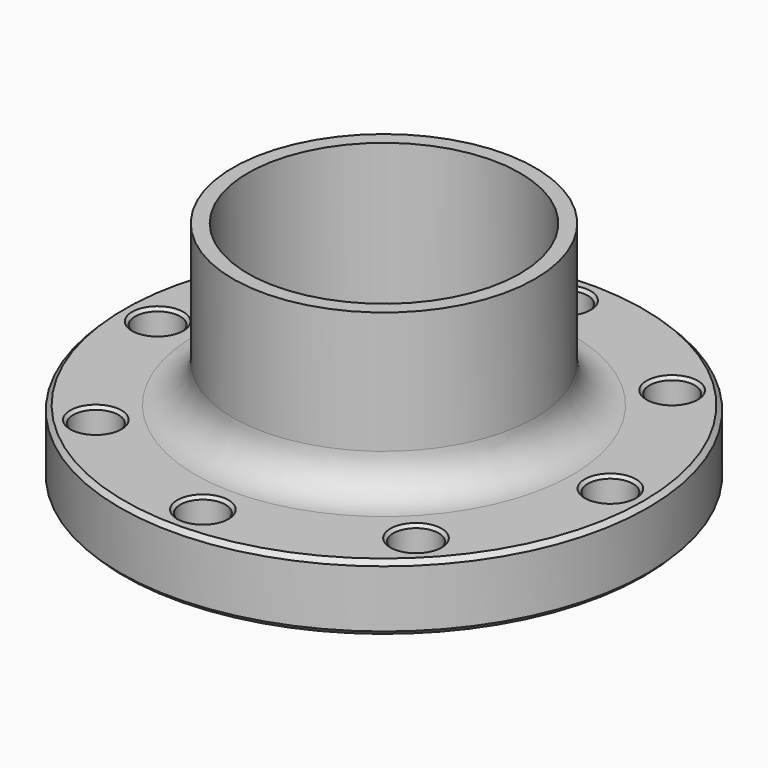
from build123d import *

# Parameters (mm, degrees)
F3_D            = 3.81
F3_CSINK_D      = 4.318
F3_CSINK_ANGLE  = 90
F3_COPIES_COUNT = 8
F4_SIZE2        = 0.381
F4_SIZE         = 0.381


# Not quite as in the source:
# - a pattern or mirror of a feature is missing from the dataset's text; its kind, count and spacing are read off the source's solid


with BuildPart() as f1:
    # F0 (on Front) → F1 (revolve)
    with BuildSketch(Plane.XZ):
        with BuildLine():
            Line((12.7, 19.05), (11.4554, 19.05))
            Line((11.4554, 19.05), (11.4554, 0))
            Line((11.4554, 0), (22.225, 0))
            Line((22.225, 0), (22.225, 5.588))
            Line((22.225, 5.588), (15.875, 5.588))
            ThreePointArc((15.875, 5.588), (13.6299359697, 6.5179359697), (12.7, 8.763))
            Line((12.7, 8.763), (12.7, 19.05))
        make_face()
    revolve(axis=Axis((0, 0, -8.7907983398), (0, 0, -1)))

    # F3 (through all)
    with Locations(Plane.XY.offset(5.588)):
        with Locations((-19.05, 0)):
            f3 = CounterSinkHole(F3_D / 2, F3_CSINK_D / 2, counter_sink_angle=F3_CSINK_ANGLE)

    # F3_copies: F3 ×8 about axis
    f3_copies_axis = Axis((0, 0, 0), (0, 0, 1))
    for i in range(1, F3_COPIES_COUNT):
        add(f3.rotate(f3_copies_axis, i * 360 / F3_COPIES_COUNT), mode=Mode.SUBTRACT)

    # F4
    f4_edges = [f1.edges().sort_by_distance(p)[0] for p in [
        (-22.225, 0, 5.588),
        (-22.225, 0, 0),
        (-11.4554, 0, 0),
    ]]
    chamfer(f4_edges, length=F4_SIZE, length2=F4_SIZE2)


solid = f1.part
